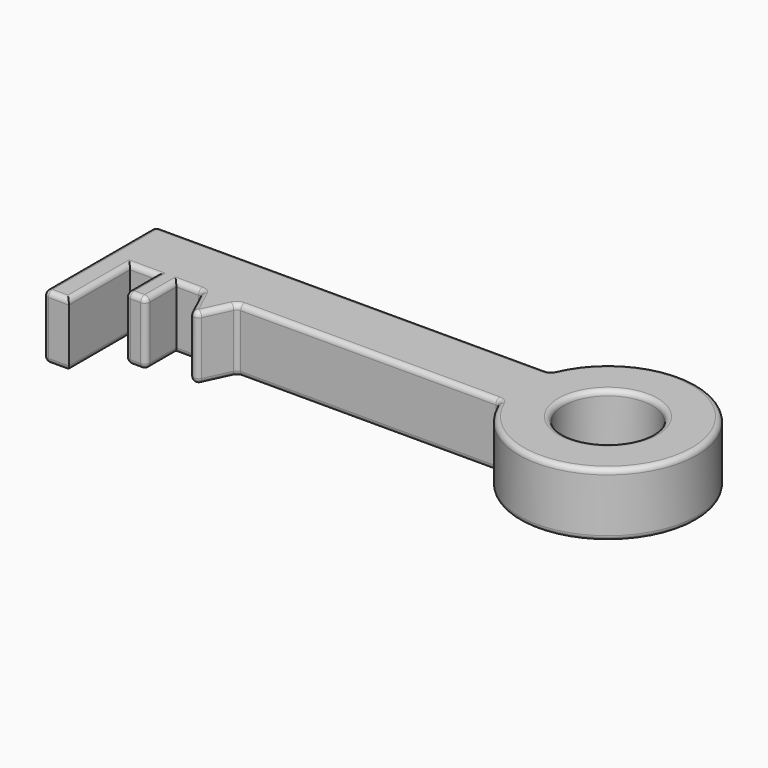
from build123d import *

# Parameters (mm, degrees)
F0_R     = 17.5
F0_W     = 10
F0_H     = 30
F0_W_2   = 8
F0_H_2   = 15
F1_DEPTH = 25
F2_R     = 2


with BuildPart() as f1:
    # F0 (on Top) → F1 (new body)
    with BuildSketch(Plane.XY):
        Polygon((77.5, -12.5), (77.5, 12.5), (-77.5, 12.5), (-77.5, -12.5), (-67.5, -12.5), (-57.2999980922, -12.5), (-49.2999980922, -12.5), (-39.2999980922, -12.5), (-25.2999980922, -12.5), align=None)
        with BuildLine():
            ThreePointArc((77.5, -12.5), (145.1917420766, 0), (77.5, 12.5))
            Line((77.5, 12.5), (77.5, -12.5))
        make_face()
        with Locations((110.1917420766, 0)):
            Circle(F0_R, mode=Mode.SUBTRACT)
        with Locations((-72.5, -27.5)):
            Rectangle(F0_W, F0_H)
        Polygon((-32.2999980922, -27.5), (-25.2999980922, -12.5), (-39.2999980922, -12.5), align=None)
        with Locations((-53.2999980922, -20)):
            Rectangle(F0_W_2, F0_H_2)
    extrude(amount=F1_DEPTH)

    # F2
    f2_edges = [f1.edges().sort_by_distance(p)[0] for p in [
        (0, 12.5, 25),
        (-77.5, -15, 25),
        (-67.5, -27.5, 25),
        (-72.5, -42.5, 25),
        (-62.399999, -12.5, 25),
        (-57.299998, -20, 25),
        (-49.299998, -20, 25),
        (-53.299998, -27.5, 25),
        (-35.799998, -20, 25),
        (26.100001, -12.5, 25),
        (-28.799998, -20, 25),
        (145.191742, 0, 25),
        (92.691742, 0, 25),
        (145.191742, 0, 0),
        (77.5, 12.5, 12.5),
        (77.5, -12.5, 12.5),
        (-77.5, 12.5, 12.5),
        (0, 12.5, 0),
        (92.691742, 0, 0),
        (26.100001, -12.5, 0),
        (-28.799998, -20, 0),
        (-44.299998, -12.5, 0),
        (-35.799998, -20, 0),
        (-49.299998, -20, 0),
        (-53.299998, -27.5, 0),
        (-57.299998, -20, 0),
        (-62.399999, -12.5, 0),
        (-67.5, -27.5, 0),
        (-77.5, -15, 0),
        (-77.5, -42.5, 12.5),
        (-32.299998, -27.5, 12.5),
        (-25.299998, -12.5, 12.5),
        (-39.299998, -12.5, 12.5),
        (-57.299998, -27.5, 12.5),
        (-49.299998, -27.5, 12.5),
        (-72.5, -42.5, 0),
        (-44.299998, -12.5, 25),
    ]]
    fillet(f2_edges, radius=F2_R)


solid = f1.part
